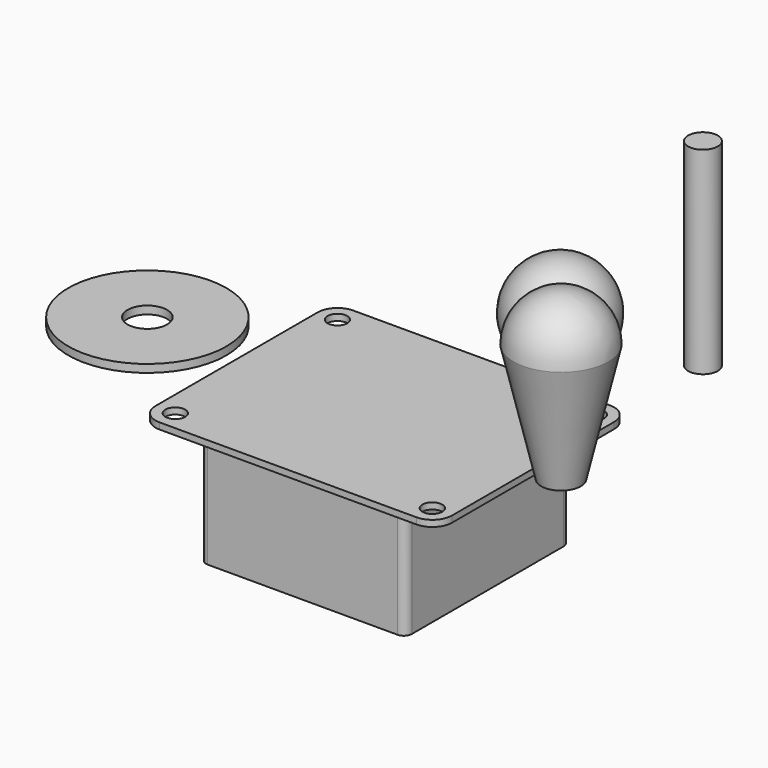
from build123d import *

# Parameters (mm, degrees)
F0_R     = 3.175
F0_R_2   = 4.7625
F1_DEPTH = 2.032
F3_DEPTH = 37.084
F8_DEPTH = 63.5
F0_R_3   = 25.4
F0_R_4   = 6.35
F9_DEPTH = 2.54


# Not quite as in the source:
# - a feature names something its author has since deleted; it is built from what else it names


with BuildPart() as f1:
    # F0 (on Top) → F1 (new body)
    with BuildSketch(Plane.XY):
        with BuildLine():
            ThreePointArc((47.625, 32.54375), (45.7651280605, 37.0338780605), (41.275, 38.89375))
            Line((41.275, 38.89375), (-41.275, 38.89375))
            ThreePointArc((-41.275, 38.89375), (-45.7651280605, 37.0338780605), (-47.625, 32.54375))
            Line((-47.625, 32.54375), (-47.625, -32.54375))
            ThreePointArc((-47.625, -32.54375), (-45.7651280605, -37.0338780605), (-41.275, -38.89375))
            Line((-41.275, -38.89375), (41.275, -38.89375))
            ThreePointArc((41.275, -38.89375), (45.7651280605, -37.0338780605), (47.625, -32.54375))
            Line((47.625, -32.54375), (47.625, 32.54375))
        make_face()
        with Locations((-41.275, -32.54375)):
            Circle(F0_R, mode=Mode.SUBTRACT)
        with Locations((41.275, -32.54375)):
            Circle(F0_R, mode=Mode.SUBTRACT)
        with Locations((-41.275, 32.54375)):
            Circle(F0_R, mode=Mode.SUBTRACT)
        Circle(F0_R_2, mode=Mode.SUBTRACT)
        with Locations((41.275, 32.54375)):
            Circle(F0_R, mode=Mode.SUBTRACT)
        Circle(F0_R_2)
    extrude(amount=-F1_DEPTH)

    # F2 (on face) → F3 (join)
    with BuildSketch(Plane(origin=(0, 0, -2.032), x_dir=(1, 0, 0), z_dir=(0, 0, -1))):
        with BuildLine():
            ThreePointArc((33.02, 30.48), (32.2760512242, 32.2760512242), (30.48, 33.02))
            Line((30.48, 33.02), (-30.48, 33.02))
            ThreePointArc((-30.48, 33.02), (-32.2760512242, 32.2760512242), (-33.02, 30.48))
            Line((-33.02, 30.48), (-33.02, -30.48))
            ThreePointArc((-33.02, -30.48), (-32.2760512242, -32.2760512242), (-30.48, -33.02))
            Line((-30.48, -33.02), (30.48, -33.02))
            ThreePointArc((30.48, -33.02), (32.2760512242, -32.2760512242), (33.02, -30.48))
            Line((33.02, -30.48), (33.02, 30.48))
        make_face()
    extrude(amount=F3_DEPTH)


with BuildPart() as f5:
    # F4 (on Top) → F5 (revolve)
    with BuildSketch(Plane.XY):
        with BuildLine():
            Line((0, 54.4698057175), (0, 86.2198057175))
            ThreePointArc((0, 86.2198057175), (-15.875, 70.3448057175), (0, 54.4698057175))
        make_face()
    revolve(axis=Axis((0, 70.3448057175, 0), (0, 1, 0)))


with BuildPart() as f7:
    # F6 (on Front) → F7 (revolve)
    with BuildSketch(Plane.XZ):
        Polygon((56.5684698522, 38.1), (56.5684698522, 0), (62.9184698522, 0), (71.8084698522, 38.1), align=None)
        with BuildLine():
            Line((56.5684698522, 53.34), (56.5684698522, 38.1))
            Line((56.5684698522, 38.1), (71.8084698522, 38.1))
            ThreePointArc((71.8084698522, 38.1), (67.3447771975, 48.8763073453), (56.5684698522, 53.34))
        make_face()
    revolve(axis=Axis((56.5684698522, 0, 19.05), (0, 0, 1)))


with BuildPart() as f8:
    # F4 (on Top) → F8 (new body)
    with BuildSketch(Plane.XY):
        with BuildLine():
            ThreePointArc((45.8889380097, 65.5823057175), (49.2565340551, 66.9772096721), (50.6514380097, 70.3448057175))
            ThreePointArc((50.6514380097, 70.3448057175), (49.2565340551, 73.7124017629), (45.8889380097, 75.1073057175))
            Line((45.8889380097, 75.1073057175), (45.8889380097, 65.5823057175))
        make_face()
        with BuildLine():
            Line((45.8889380097, 65.5823057175), (45.8889380097, 75.1073057175))
            ThreePointArc((45.8889380097, 75.1073057175), (41.1264380097, 70.3448057175), (45.8889380097, 65.5823057175))
        make_face()
    extrude(amount=F8_DEPTH)


with BuildPart() as f9:
    # F0 (on Top) → F9 (new body)
    with BuildSketch(Plane.XY):
        with Locations((-76.2901902199, 0)):
            Circle(F0_R_3)
        with Locations((-76.2901902199, 0)):
            Circle(F0_R_4, mode=Mode.SUBTRACT)
    extrude(amount=F9_DEPTH)


solid = Compound([f1.part, f5.part, f7.part, f8.part, f9.part])
